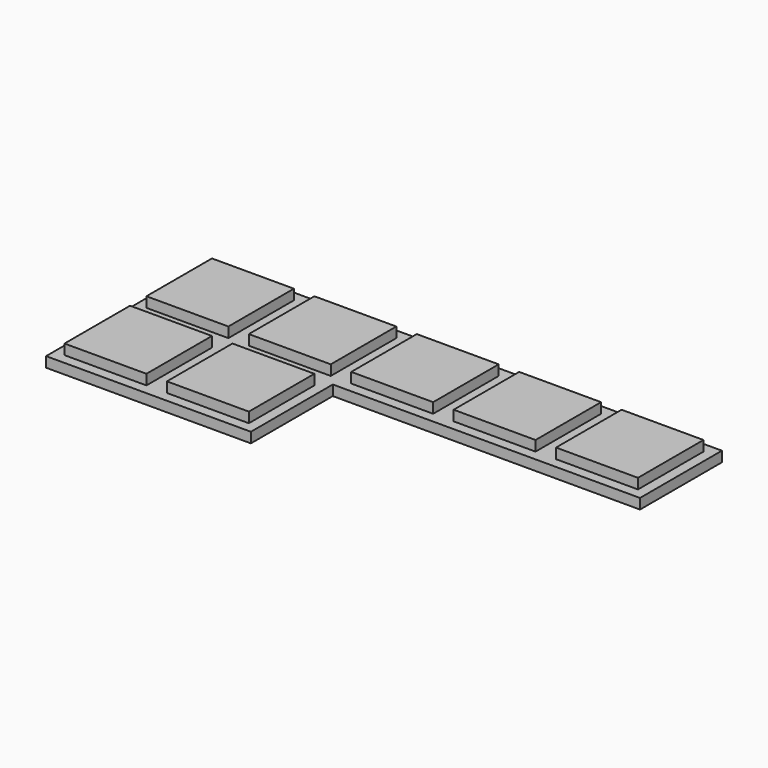
from build123d import *

# Parameters (mm, degrees)
F1_DEPTH = 1
F2_W     = 8
F2_H     = 8
F3_DEPTH = 1


# Not quite as in the source:
# - a feature names something its author has since deleted; it is built from what else it names


with BuildPart() as f1:
    # F0 (on Top) → F1 (new body)
    with BuildSketch(Plane.XY):
        Polygon((30, 10), (-20, 10), (-20, -10), (0, -10), (0, 0), (30, 0), align=None)
    extrude(amount=F1_DEPTH)

    # F2 (on face) → F3 (join)
    with BuildSketch(Plane.XY.offset(1)):
        with Locations((-15, 5)):
            Rectangle(F2_W, F2_H)
        with Locations((-15, -5)):
            Rectangle(F2_W, F2_H)
        with Locations((-5, -5)):
            Rectangle(F2_W, F2_H)
        with Locations((-5, 5)):
            Rectangle(F2_W, F2_H)
        with Locations((5, 5)):
            Rectangle(F2_W, F2_H)
        with Locations((15, 5)):
            Rectangle(F2_W, F2_H)
        with Locations((25, 5)):
            Rectangle(F2_W, F2_H)
    extrude(amount=F3_DEPTH)


solid = f1.part
